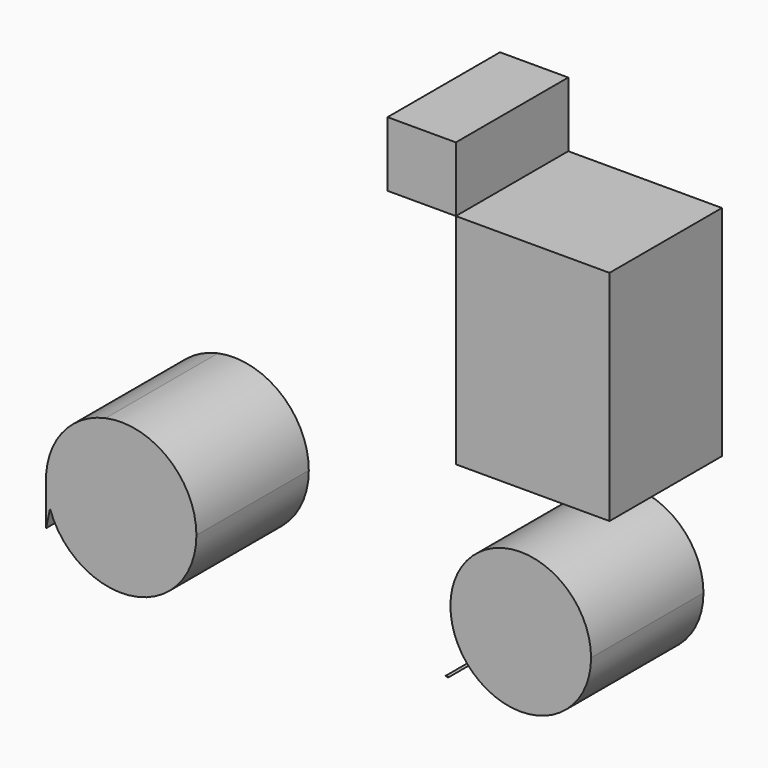
from build123d import *

# Parameters (mm, degrees)
F1_DEPTH = 12.446
F0_W     = 6.0499049723
F0_H     = 5.7474076748
F0_W_2   = 13.612287119
F0_H_2   = 19.3596985191


with BuildPart() as f1:
    # F0 (on Front) → F1 (new body)
    with BuildSketch(Plane.XZ):
        with BuildLine():
            Line((-49.9117225409, 3.4786572239), (-49.9117225409, 0))
            add(Edge.make_bspline(
                [(-49.5652059441, 1.6402761529), (-49.6836660494, 1.09742076), (-49.7976942951, 0.54871038), (-49.9117225409, 0)],
                knots=[0.9495226435, 0.9495226435, 0.9495226435, 0.9495226435, 1, 1, 1, 1], degree=3))
            ThreePointArc((-49.5652059441, 1.6402761529), (-49.8033170935, 2.5472425692), (-49.9117225409, 3.4786572239))
        make_face()
        with BuildLine():
            ThreePointArc((-49.9117225409, 4.0837249228), (-49.918595638, 3.7811910734), (-49.9117225409, 3.4786572239))
            Line((-49.9117225409, 3.4786572239), (-49.9117225409, 4.0837249228))
        make_face()
        with BuildLine():
            Line((-49.9117225409, 4.0837249228), (-49.9117225409, 3.4786572239))
            ThreePointArc((-49.9117225409, 3.4786572239), (-49.8033170935, 2.5472425692), (-49.5652059441, 1.6402761529))
            add(Edge.make_bspline(
                [(-44.6397836083, 10.2978309733), (-45.119653972, 10.1041501862), (-47.8014157398, 8.582874138), (-48.8523363966, 4.9070728269), (-49.5652059441, 1.6402761529)],
                knots=[0.584004576, 0.584004576, 0.584004576, 0.584004576, 0.6457598692, 0.9495226435, 0.9495226435, 0.9495226435, 0.9495226435], degree=3))
            ThreePointArc((-44.6397836083, 10.2978309733), (-48.3367428118, 8.090903092), (-49.9117225409, 4.0837249228))
        make_face()
        with BuildLine():
            add(Edge.make_bspline(
                [(-44.6397836083, 10.2978309733), (-45.119653972, 10.1041501862), (-47.8014157398, 8.582874138), (-48.8523363966, 4.9070728269), (-49.5652059441, 1.6402761529)],
                knots=[0.584004576, 0.584004576, 0.584004576, 0.584004576, 0.6457598692, 0.9495226435, 0.9495226435, 0.9495226435, 0.9495226435], degree=3))
            ThreePointArc((-49.5652059441, 1.6402761529), (-42.171884192, -2.7916367166), (-36.5950577596, 3.7811910734))
            ThreePointArc((-36.5950577596, 3.7811910734), (-39.0636044286, 8.957681428), (-44.6397836083, 10.2978309733))
        make_face()
    extrude(amount=F1_DEPTH)


with BuildPart() as f1b:
    # F0 (on Front) → F1, piece 2 (new body)
    with BuildSketch(Plane.XZ):
        with Locations((-16.6372396052, 39.0218906105)):
            Rectangle(F0_W, F0_H)
    extrude(amount=F1_DEPTH)


with BuildPart() as f1c:
    # F0 (on Front) → F1, piece 3 (new body)
    with BuildSketch(Plane.XZ):
        with BuildLine():
            Line((-14.2172779888, 0), (-14.5197734237, 0))
            add(Edge.make_bspline(
                [(-14.2172779888, 0), (-14.3061968444, -0.0872909317), (-14.412985134, -0.0436454659), (-14.5197734237, 0)],
                knots=[0.952469801, 0.952469801, 0.952469801, 0.952469801, 1, 1, 1, 1], degree=3))
        make_face()
    extrude(amount=F1_DEPTH)


with BuildPart() as f1d:
    # F0 (on Front) → F1, piece 4 (new body)
    with BuildSketch(Plane.XZ):
        with Locations((-6.8061435595, 26.4683375135)):
            Rectangle(F0_W_2, F0_H_2)
    extrude(amount=F1_DEPTH)


with BuildPart() as f1e:
    # F0 (on Front) → F1, piece 5 (new body)
    with BuildSketch(Plane.XZ):
        with BuildLine():
            ThreePointArc((-13.0991596694, 8.9725089924), (-14.0512340104, 6.3217092663), (-13.7383403252, 3.5225518431))
            add(Edge.make_bspline(
                [(-13.0991596694, 8.9725089924), (-13.4021570242, 7.995667339), (-13.5891754167, 6.2309110491), (-13.6990528868, 4.2034320829), (-13.7383403252, 3.5225518431)],
                knots=[0.6405219867, 0.6405219867, 0.6405219867, 0.6405219867, 0.7474400174, 0.8053833563, 0.8053833563, 0.8053833563, 0.8053833563], degree=3))
        make_face()
        with BuildLine():
            add(Edge.make_bspline(
                [(-13.0991596694, 8.9725089924), (-13.4021570242, 7.995667339), (-13.5891754167, 6.2309110491), (-13.6990528868, 4.2034320829), (-13.7383403252, 3.5225518431)],
                knots=[0.6405219867, 0.6405219867, 0.6405219867, 0.6405219867, 0.7474400174, 0.8053833563, 0.8053833563, 0.8053833563, 0.8053833563], degree=3))
            ThreePointArc((-13.7383403252, 3.5225518431), (-6.8129623392, -0.5431301891), (-1.6361178808, 5.5961622857))
            ThreePointArc((-1.6361178808, 5.5961622857), (-6.1049974568, 11.5711318281), (-13.0991596694, 8.9725089924))
        make_face()
    extrude(amount=F1_DEPTH)


solid = Compound([f1.part, f1b.part, f1c.part, f1d.part, f1e.part])
